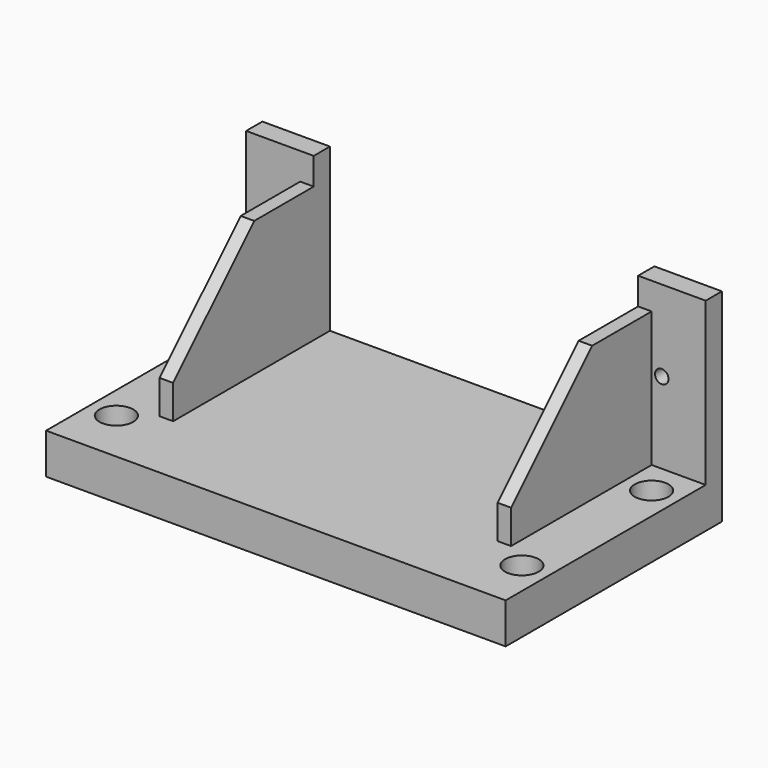
from build123d import *

# Parameters (mm, degrees)
F0_W     = 34
F0_H     = 20
F0_R     = 1.25
F1_DEPTH = 3
F2_W     = 5
F2_H     = 1.5
F3_DEPTH = 12
F4_W     = 1
F4_H     = 13
F5_DEPTH = 10
F6_SIZE  = 7.5
F8_D     = 1


# Not quite as in the source:
# - a feature names something its author has since deleted; it is built from what else it names


with BuildPart() as f1:
    # F0 (on Top) → F1 (new body)
    with BuildSketch(Plane.XY):
        Rectangle(F0_W, F0_H)
        with Locations((-15, -6)):
            Circle(F0_R, mode=Mode.SUBTRACT)
        with Locations((15, -6)):
            Circle(F0_R, mode=Mode.SUBTRACT)
        with Locations((-15, 6)):
            Circle(F0_R, mode=Mode.SUBTRACT)
        with Locations((15, 6)):
            Circle(F0_R, mode=Mode.SUBTRACT)
    extrude(amount=F1_DEPTH)

    # F2 (on face) → F3 (join)
    with BuildSketch(Plane.XY.offset(3)):
        with Locations((-14.5, 9.25)):
            Rectangle(F2_W, F2_H)
        with Locations((14.5, 9.25)):
            Rectangle(F2_W, F2_H)
    extrude(amount=F3_DEPTH)

    # F4 (on face) → F5 (join)
    with BuildSketch(Plane.XY.offset(3)):
        with Locations((-12.5, 2)):
            Rectangle(F4_W, F4_H)
        with Locations((12.5, 2)):
            Rectangle(F4_W, F4_H)
    extrude(amount=F5_DEPTH)

    # F6
    f6_edges = [f1.edges().sort_by_distance(p)[0] for p in [
        (-12.5, -4.5, 13),
        (12.5, -4.5, 13),
    ]]
    chamfer(f6_edges, length=F6_SIZE)

    # F8 (through all)
    with Locations(Plane(origin=(0, 10, 0), x_dir=(-1, 0, 0), z_dir=(0, 1, 0))):
        with Locations((13.75, 9), (-13.75, 9)):
            Hole(F8_D / 2)


solid = f1.part
